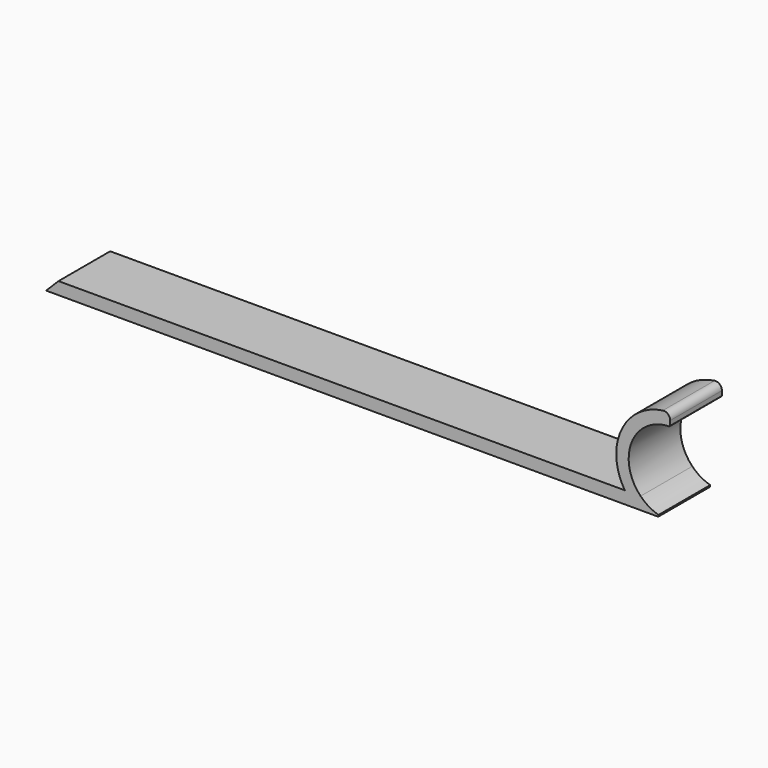
from build123d import *

# Parameters (mm, degrees)
F1_DEPTH    = 15
F2_T1_DEPTH = 28.8982001462
F2_T3_DEPTH = 16.0188013663
F3_T1_DEPTH = 30.3272306083
F4_R        = 1.5


# Not quite as in the source:
# - a fillet or chamfer that OpenCascade refuses, or shapes differently, is made with other operations: its cross-section is extruded or revolved along the edge and cut away or added
# - a feature names something its author has since deleted; it is built from what else it names


with BuildPart() as f1:
    # F0 (on Front) → F1 (new body)
    with BuildSketch(Plane.XZ):
        with BuildLine():
            ThreePointArc((64.5076036134, -1.44), (63.120788421, -0.0985070956), (61.9563763345, 1.44))
            Line((61.9563763345, 1.44), (-72.5, 1.44))
            Line((-72.5, 1.44), (-72.5, -1.44))
            Line((-72.5, -1.44), (64.5076036134, -1.44))
        make_face()
        with BuildLine():
            Line((61.9563763345, 1.44), (65.6232565847, 1.44))
            ThreePointArc((65.6232565847, 1.44), (63.599073082, 11.9377338961), (72.5, 17.86))
            Line((72.5, 17.86), (72.5, 20.74))
            ThreePointArc((72.5, 20.74), (61.5038870504, 14.2171956852), (61.9563763345, 1.44))
        make_face()
        with BuildLine():
            ThreePointArc((72.5, -1.44), (68.7722661039, -0.690926918), (65.6232565847, 1.44))
            Line((65.6232565847, 1.44), (61.9563763345, 1.44))
            ThreePointArc((61.9563763345, 1.44), (63.120788421, -0.0985070956), (64.5076036134, -1.44))
            Line((64.5076036134, -1.44), (72.5, -1.44))
        make_face()
    extrude(amount=F1_DEPTH)

    # F2: chamfer of 0.2 on 2 edges, made by hand

    # F2_s2 → F2_t1 (cut)
    with BuildSketch(Plane.XZ.offset(-6.9491000731)):
        with BuildLine():
            Line((69.7215112021, -1.44), (69.7779272183, -1.0481218274))
            ThreePointArc((69.7779272183, -1.0481218274), (71.1249319352, -1.3415280357), (72.5, -1.44))
            Line((72.5, -1.44), (69.7215112021, -1.44))
        make_face()
    extrude(amount=F2_T1_DEPTH, mode=Mode.SUBTRACT)

    # F2_s4 → F2_t3 (cut)
    with BuildSketch(Plane.XZ.offset(-0.5094006831)):
        with BuildLine():
            Line((72.3040609137, 17.8580105656), (72.5, 18.0579693338))
            Line((72.5, 18.0579693338), (72.5, 17.86))
            ThreePointArc((72.5, 17.86), (72.399196155, 17.8594734874), (72.3040609137, 17.8580105656))
        make_face()
    extrude(amount=F2_T3_DEPTH, mode=Mode.SUBTRACT)

    # F3: chamfer of 2.98 on 1 edges, made by hand

    # F3_s2 → F3_t1 (cut)
    with BuildSketch(Plane.XZ.offset(-7.6636153041)):
        Polygon((-72.5, -1.54), (-69.52, 1.44), (-72.5, 1.44), align=None)
    extrude(amount=F3_T1_DEPTH, mode=Mode.SUBTRACT)

    # F4
    f4_edges = [f1.edges().sort_by_distance(p)[0] for p in [
        (72.5, -7.5, 20.74),
    ]]
    fillet(f4_edges, radius=F4_R)


solid = f1.part
